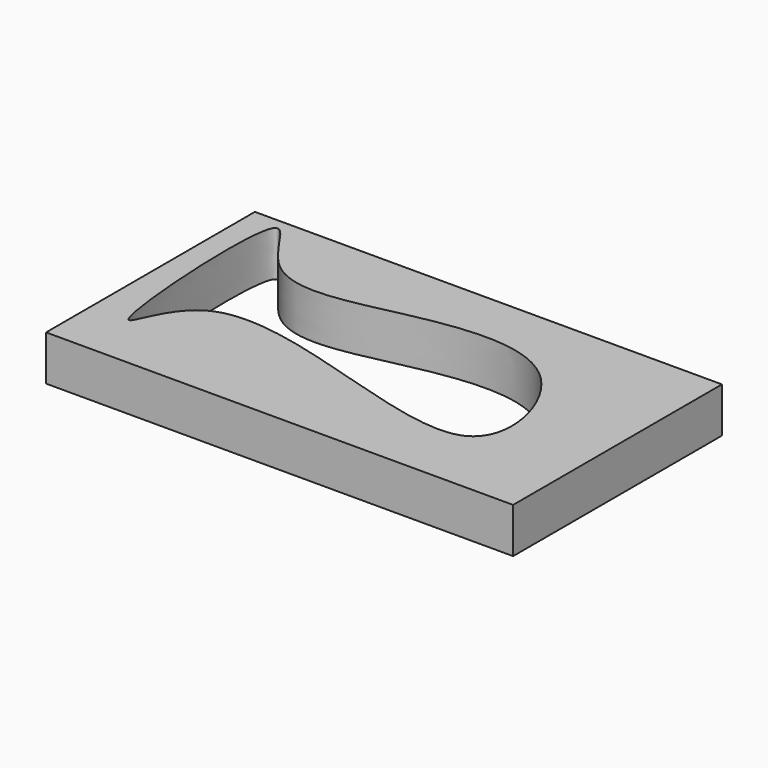
from build123d import *

# Parameters (mm, degrees)
F0_W     = 262.832909
F0_H     = 146.897569
F1_DEPTH = 25.4
F3_DEPTH = 25.401


with BuildPart() as f1:
    # F0 (on Top) → F1 (new body)
    with BuildSketch(Plane.XY):
        with Locations((6.660908, 7.559136)):
            Rectangle(F0_W, F0_H)
    extrude(amount=F1_DEPTH)

    # F2 (on face) → F3 (cut, through all)
    with BuildSketch(Plane.XY.offset(25.4)):
        with BuildLine():
            add(Edge.make_bspline(
                [(-81.264846, -4.941447), (-45.65308, 12.476917), (113.321807, -76.79323), (79.668553, 60.028693), (-10.782863, 49.100258), (-84.181839, 26.307152), (-119.158762, 117.697585), (-106.133596, -79.447067), (-98.11394, -13.182646), (-81.264846, -4.941447)],
                knots=[0, 0, 0, 0, 0.20978, 0.341425, 0.491241, 0.630601, 0.730658, 0.900746, 1, 1, 1, 1], degree=3))
        make_face()
    extrude(amount=-F3_DEPTH, mode=Mode.SUBTRACT)


solid = f1.part
